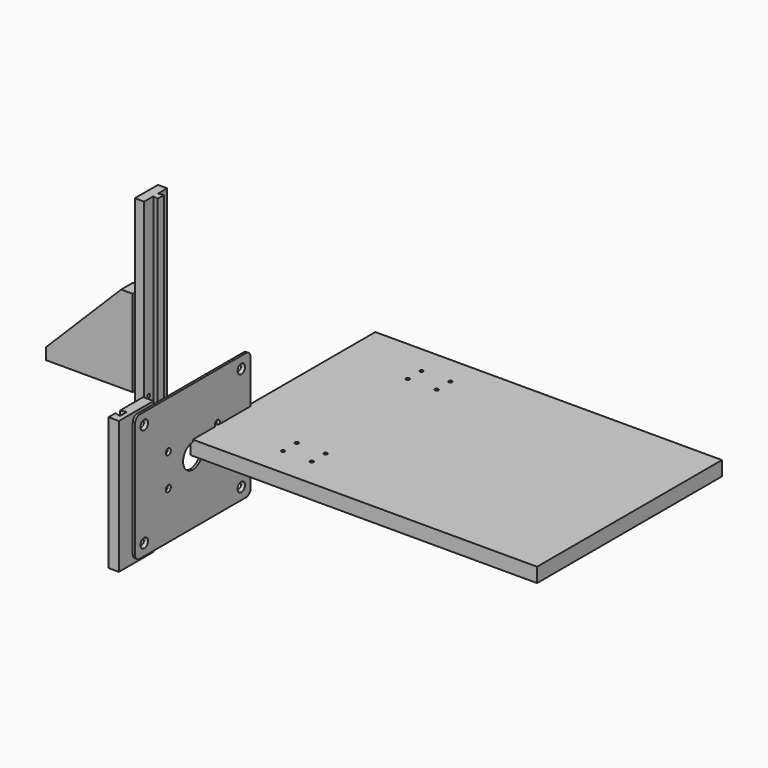
from build123d import *

# Parameters (mm, degrees)
F0_R      = 4.125
F0_R_2    = 2.5
F0_R_3    = 21
F1_DEPTH  = 4
F2_SIZE   = 3.99999
F3_SIZE   = 3
F4_W      = 75
F4_H      = 230
F4_R      = 4.125
F5_DEPTH  = 18
F7_DEPTH  = 230
F8_R      = 10
F9_DEPTH  = 20
F11_DEPTH = 400
F12_R     = 3
F13_DEPTH = 25
F14_R     = 5
F15_DEPTH = 12
F18_W     = 600
F18_H     = 400
F18_R     = 3
F19_DEPTH = 25
F21_DEPTH = 25
F22_R     = 3
F23_DEPTH = 35
F24_R     = 3
F25_DEPTH = 35


# Not quite as in the source:
# - a fillet or chamfer is up to 0.001 mm smaller than in the source, because OpenCascade refuses the exact size


with BuildPart() as f1:
    # F0 (on Right) → F1 (new body)
    with BuildSketch(Plane.YZ):
        with BuildLine():
            Line((115, 110), (-115, 110))
            ThreePointArc((-115, 110), (-122.0710678119, 107.0710678119), (-125, 100))
            Line((-125, 100), (-125, -100))
            ThreePointArc((-125, -100), (-122.0710678119, -107.0710678119), (-115, -110))
            Line((-115, -110), (115, -110))
            ThreePointArc((115, -110), (122.0710678119, -107.0710678119), (125, -100))
            Line((125, -100), (125, 100))
            ThreePointArc((125, 100), (122.0710678119, 107.0710678119), (115, 110))
        make_face()
        with Locations((-105, -90)):
            Circle(F0_R, mode=Mode.SUBTRACT)
        with Locations((-53, -28)):
            Circle(F0_R_2, mode=Mode.SUBTRACT)
        with Locations((105, -90)):
            Circle(F0_R, mode=Mode.SUBTRACT)
        with Locations((53, -28)):
            Circle(F0_R_2, mode=Mode.SUBTRACT)
        with Locations((-53, 28)):
            Circle(F0_R_2, mode=Mode.SUBTRACT)
        with Locations((-105, 90)):
            Circle(F0_R, mode=Mode.SUBTRACT)
        Circle(F0_R_3, mode=Mode.SUBTRACT)
        with Locations((53, 28)):
            Circle(F0_R_2, mode=Mode.SUBTRACT)
        with Locations((105, 90)):
            Circle(F0_R, mode=Mode.SUBTRACT)
    extrude(amount=F1_DEPTH)

    # F2 (size 4 in the source; OpenCascade refuses exactly that, so slightly less here)
    f2_edges = [f1.edges().sort_by_distance(p)[0] for p in [
        (4, -109.125, 90),
        (4, 100.875, 90),
        (4, 100.875, -90),
        (4, -109.125, -90),
    ]]
    chamfer(f2_edges, length=F2_SIZE)

    # F3
    f3_edges = [f1.edges().sort_by_distance(p)[0] for p in [
        (4, -55.5, 28),
        (4, -55.5, -28),
        (4, 50.5, -28),
        (4, 50.5, 28),
    ]]
    chamfer(f3_edges, length=F3_SIZE)


with BuildPart() as f5:
    # F4 (on face) → F5 (new body)
    with BuildSketch(Plane(origin=(0, 0, 0), x_dir=(0, -1, 0), z_dir=(-1, 0, 0))):
        with Locations((117.5, 0)):
            Rectangle(F4_W, F4_H)
        with Locations((105, -90)):
            Circle(F4_R, mode=Mode.SUBTRACT)
        with Locations((105, 90)):
            Circle(F4_R, mode=Mode.SUBTRACT)
    extrude(amount=F5_DEPTH)

    # F6 (on face) → F7 (cut, through all)
    with BuildSketch(Plane.XY.offset(115)):
        Polygon((-18, -130), (-18, -140.0134399431), (-8, -142.5067199716), (-8, -127.5067199716), align=None)
    extrude(amount=-F7_DEPTH, mode=Mode.SUBTRACT)

    # F8 (on face) → F9 (join)
    with BuildSketch(Plane(origin=(-18, 0, 0), x_dir=(0, -1, 0), z_dir=(-1, 0, 0))):
        with Locations((95, 0)):
            Circle(F8_R)
    extrude(amount=F9_DEPTH)


with BuildPart() as f11:
    # F10 (on Top) → F11 (new body)
    with BuildSketch(Plane.XY):
        Polygon((-48.6005372249, -59.6890420537), (-32.6005372249, -59.6890420537), (-32.6005372249, -39.6890420537), (-23.6005372249, -41.9329940793), (-23.6005372249, -27.4450900281), (-32.6005372249, -29.6890420537), (-32.6005372249, -9.6890420537), (-48.6005372249, -9.6890420537), align=None)
    extrude(amount=F11_DEPTH)

    # F12 (on face) → F13 (cut)
    with BuildSketch(Plane(origin=(-48.6005372249, 0, 0), x_dir=(0, -1, 0), z_dir=(-1, 0, 0))):
        with Locations((49.6890420537, 50)):
            Circle(F12_R)
        with Locations((49.6890420537, 100)):
            Circle(F12_R)
        with Locations((19.6890420537, 100)):
            Circle(F12_R)
        with Locations((19.6890420537, 50)):
            Circle(F12_R)
    extrude(amount=-F13_DEPTH, mode=Mode.SUBTRACT)

    # F14 (on face) → F15 (join)
    with BuildSketch(Plane(origin=(-48.6005372249, 0, 0), x_dir=(0, -1, 0), z_dir=(-1, 0, 0))):
        with Locations((34.6890420537, 375)):
            Circle(F14_R)
    extrude(amount=F15_DEPTH)


with BuildPart() as f17:
    # F16 (on Top) → F17 (revolve)
    with BuildSketch(Plane.XY):
        Polygon((-62.5817395097, 57.1463547086), (-62.5817395097, 29.1463547086), (-58.5817395097, 29.1463547086), (-58.5817395097, 57.1463547086), (-55.5817395097, 61.1463547086), (-55.5817395097, 69.1463547086), (-58.0817395097, 69.1463547086), (-59.3317395097, 66.1463547086), (-61.8317395097, 66.1463547086), (-63.0817395097, 69.1463547086), (-65.5817395097, 69.1463547086), (-65.5817395097, 61.1463547086), align=None)
    revolve(axis=Axis((-60.5817395097, 24.1463547086, 0), (1, 0, 0)))


with BuildPart() as f19:
    # F18 (on Top) → F19 (new body)
    with BuildSketch(Plane.XY):
        with Locations((300, 200)):
            Rectangle(F18_W, F18_H)
        with Locations((120, 50)):
            Circle(F18_R, mode=Mode.SUBTRACT)
        with Locations((120, 80)):
            Circle(F18_R, mode=Mode.SUBTRACT)
        with Locations((170, 50)):
            Circle(F18_R, mode=Mode.SUBTRACT)
        with Locations((170, 80)):
            Circle(F18_R, mode=Mode.SUBTRACT)
        with Locations((120, 320)):
            Circle(F18_R, mode=Mode.SUBTRACT)
        with Locations((120, 350)):
            Circle(F18_R, mode=Mode.SUBTRACT)
        with Locations((170, 320)):
            Circle(F18_R, mode=Mode.SUBTRACT)
        with Locations((170, 350)):
            Circle(F18_R, mode=Mode.SUBTRACT)
    extrude(amount=F19_DEPTH)


with BuildPart() as f21:
    # F20 (on Front) → F21 (new body)
    with BuildSketch(Plane.XZ):
        Polygon((-230, 80), (-80, 80), (-80, 230), (-100, 230), (-230, 100), align=None)
    extrude(amount=F21_DEPTH)

    # F22 (on face) → F23 (cut)
    with BuildSketch(Plane(origin=(0, 0, 80), x_dir=(1, 0, 0), z_dir=(0, 0, -1))):
        with Locations((-180, 12.5)):
            Circle(F22_R)
        with Locations((-130, 12.5)):
            Circle(F22_R)
    extrude(amount=-F23_DEPTH, mode=Mode.SUBTRACT)

    # F24 (on face) → F25 (cut)
    with BuildSketch(Plane.YZ.offset(-80)):
        with Locations((-12.5, 180)):
            Circle(F24_R)
        with Locations((-12.5, 130)):
            Circle(F24_R)
    extrude(amount=-F25_DEPTH, mode=Mode.SUBTRACT)


solid = Compound([f1.part, f5.part, f11.part, f17.part, f19.part, f21.part])
